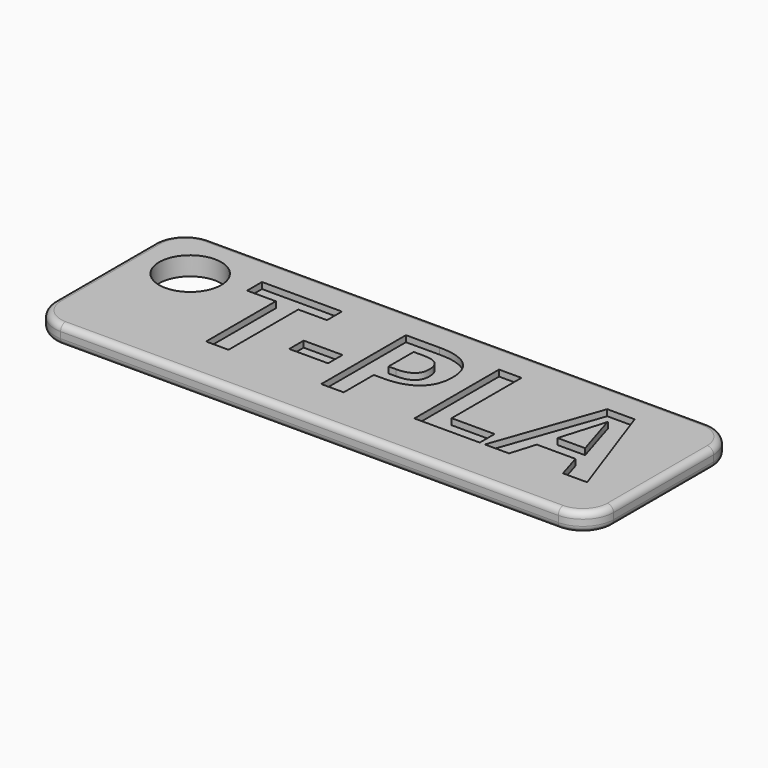
from build123d import *

# Parameters (mm, degrees)
F0_W         = 90
F0_H         = 30
F1_DEPTH     = 3
F2_R         = 1
F3_T1_DEPTH  = 3
F3_T4_ANGLE  = 90
F3_T6_ANGLE  = 90
F3_T8_ANGLE  = 90
F3_T10_ANGLE = 90
F3_T12_ANGLE = 90
F3_T14_ANGLE = 90
F3_T16_ANGLE = 90
F3_T18_ANGLE = 90
F4_R         = 5
F5_DEPTH     = 3
F6_TEXT_SIZE = 23.8714277878
F7_DEPTH     = 1


# Not quite as in the source:
# - a fillet or chamfer that OpenCascade refuses, or shapes differently, is made with other operations: its cross-section is extruded or revolved along the edge and cut away or added
# - Text() gives the source's letters only with a copy of the font that has no kerning and outlines rounded to 1/6400 em; it was checked with that copy


with BuildPart() as f1:
    # F0 (on Top) → F1 (new body)
    with BuildSketch(Plane.XY):
        Rectangle(F0_W, F0_H)
    extrude(amount=F1_DEPTH)

    # F2
    f2_edges = [f1.edges().sort_by_distance(p)[0] for p in [
        (0, 15, 3),
        (-45, 0, 3),
        (0, -15, 3),
        (45, 0, 3),
        (0, 15, 0),
        (-45, 0, 0),
        (0, -15, 0),
        (45, 0, 0),
    ]]
    fillet(f2_edges, radius=F2_R)

    # F3: fillet of radius 5 on 4 edges, made by hand

    # F3_s2 → F3_t1 (cut)
    with BuildSketch(Plane.XY):
        with BuildLine():
            ThreePointArc((45.0004, -9.9990343146), (43.5355339059, -13.5355339059), (39.9990343146, -15.0004))
            Line((39.9990343146, -15.0004), (39.9990343146, -15.5005365685))
            ThreePointArc((39.9990343146, -15.5005365685), (42.4995171573, -15.5001365685), (45, -15.5001365685))
            Line((45, -15.5001365685), (45.5001365685, -15))
            ThreePointArc((45.5001365685, -15), (45.5001365685, -12.4995171573), (45.5005365685, -9.9990343146))
            Line((45.5005365685, -9.9990343146), (45.0004, -9.9990343146))
        make_face()
        with BuildLine():
            ThreePointArc((39.9990343146, 15.0004), (43.5355339059, 13.5355339059), (45.0004, 9.9990343146))
            Line((45.0004, 9.9990343146), (45.5005365685, 9.9990343146))
            ThreePointArc((45.5005365685, 9.9990343146), (45.5001365685, 12.4995171573), (45.5001365685, 15))
            Line((45.5001365685, 15), (45, 15.5001365685))
            ThreePointArc((45, 15.5001365685), (42.4995171573, 15.5001365685), (39.9990343146, 15.5005365685))
            Line((39.9990343146, 15.5005365685), (39.9990343146, 15.0004))
        make_face()
        with BuildLine():
            ThreePointArc((-39.9990343146, 15.0004), (-43.5355339059, 13.5355339059), (-45.0004, 9.9990343146))
            Line((-45.0004, 9.9990343146), (-45.5005365685, 9.9990343146))
            ThreePointArc((-45.5005365685, 9.9990343146), (-45.5001365685, 12.4995171573), (-45.5001365685, 15))
            Line((-45.5001365685, 15), (-45, 15.5001365685))
            ThreePointArc((-45, 15.5001365685), (-42.4995171573, 15.5001365685), (-39.9990343146, 15.5005365685))
            Line((-39.9990343146, 15.5005365685), (-39.9990343146, 15.0004))
        make_face()
        with BuildLine():
            ThreePointArc((-45.0004, -9.9990343146), (-43.5355339059, -13.5355339059), (-39.9990343146, -15.0004))
            Line((-39.9990343146, -15.0004), (-39.9990343146, -15.5005365685))
            ThreePointArc((-39.9990343146, -15.5005365685), (-42.4995171573, -15.5001365685), (-45, -15.5001365685))
            Line((-45, -15.5001365685), (-45.5001365685, -15))
            ThreePointArc((-45.5001365685, -15), (-45.5001365685, -12.4995171573), (-45.5005365685, -9.9990343146))
            Line((-45.5005365685, -9.9990343146), (-45.0004, -9.9990343146))
        make_face()
    extrude(amount=F3_T1_DEPTH, mode=Mode.SUBTRACT)

    # F3_s3 → F3_t4 (revolve, cut)
    with BuildSketch(Plane.YZ.offset(-39.9990343146)):
        with BuildLine():
            ThreePointArc((-14.0004, 0), (-14.7075067812, 0.2928932188), (-15.0004, 1))
            Line((-15.0004, 1), (-15.0004, 0))
            Line((-15.0004, 0), (-14.0004, 0))
        make_face()
    revolve(axis=Axis((-39.9990343146, -9.9990343146, 0), (0, 0, -1)), revolution_arc=F3_T4_ANGLE, mode=Mode.SUBTRACT)

    # F3_s5 → F3_t6 (revolve, cut)
    with BuildSketch(Plane.XZ.offset(9.9990343146)):
        with BuildLine():
            ThreePointArc((-44.0004, 3), (-44.7075067812, 2.7071067812), (-45.0004, 2))
            Line((-45.0004, 2), (-45.0004, 3))
            Line((-45.0004, 3), (-44.0004, 3))
        make_face()
    revolve(axis=Axis((-39.9990343146, -9.9990343146, 3), (0, 0, 1)), revolution_arc=F3_T6_ANGLE, mode=Mode.SUBTRACT)

    # F3_s7 → F3_t8 (revolve, cut)
    with BuildSketch(Plane.XZ.offset(-9.9990343146)):
        with BuildLine():
            ThreePointArc((-44.0004, 0), (-44.7075067812, 0.2928932188), (-45.0004, 1))
            Line((-45.0004, 1), (-45.0004, 0))
            Line((-45.0004, 0), (-44.0004, 0))
        make_face()
    revolve(axis=Axis((-39.9990343146, 9.9990343146, 0), (0, 0, -1)), revolution_arc=F3_T8_ANGLE, mode=Mode.SUBTRACT)

    # F3_s9 → F3_t10 (revolve, cut)
    with BuildSketch(Plane.YZ.offset(-39.9990343146)):
        with BuildLine():
            ThreePointArc((14.0004, 3), (14.7075067812, 2.7071067812), (15.0004, 2))
            Line((15.0004, 2), (15.0004, 3))
            Line((15.0004, 3), (14.0004, 3))
        make_face()
    revolve(axis=Axis((-39.9990343146, 9.9990343146, 3), (0, 0, 1)), revolution_arc=F3_T10_ANGLE, mode=Mode.SUBTRACT)

    # F3_s11 → F3_t12 (revolve, cut)
    with BuildSketch(Plane.YZ.offset(39.9990343146)):
        with BuildLine():
            ThreePointArc((14.0004, 0), (14.7075067812, 0.2928932188), (15.0004, 1))
            Line((15.0004, 1), (15.0004, 0))
            Line((15.0004, 0), (14.0004, 0))
        make_face()
    revolve(axis=Axis((39.9990343146, 9.9990343146, 0), (0, 0, -1)), revolution_arc=F3_T12_ANGLE, mode=Mode.SUBTRACT)

    # F3_s13 → F3_t14 (revolve, cut)
    with BuildSketch(Plane.XZ.offset(-9.9990343146)):
        with BuildLine():
            ThreePointArc((44.0004, 3), (44.7075067812, 2.7071067812), (45.0004, 2))
            Line((45.0004, 2), (45.0004, 3))
            Line((45.0004, 3), (44.0004, 3))
        make_face()
    revolve(axis=Axis((39.9990343146, 9.9990343146, 3), (0, 0, 1)), revolution_arc=F3_T14_ANGLE, mode=Mode.SUBTRACT)

    # F3_s15 → F3_t16 (revolve, cut)
    with BuildSketch(Plane.XZ.offset(9.9990343146)):
        with BuildLine():
            ThreePointArc((44.0004, 0), (44.7075067812, 0.2928932188), (45.0004, 1))
            Line((45.0004, 1), (45.0004, 0))
            Line((45.0004, 0), (44.0004, 0))
        make_face()
    revolve(axis=Axis((39.9990343146, -9.9990343146, 0), (0, 0, -1)), revolution_arc=F3_T16_ANGLE, mode=Mode.SUBTRACT)

    # F3_s17 → F3_t18 (revolve, cut)
    with BuildSketch(Plane.YZ.offset(39.9990343146)):
        with BuildLine():
            ThreePointArc((-14.0004, 3), (-14.7075067812, 2.7071067812), (-15.0004, 2))
            Line((-15.0004, 2), (-15.0004, 3))
            Line((-15.0004, 3), (-14.0004, 3))
        make_face()
    revolve(axis=Axis((39.9990343146, -9.9990343146, 3), (0, 0, 1)), revolution_arc=F3_T18_ANGLE, mode=Mode.SUBTRACT)

    # F4 (on face) → F5 (cut)
    with BuildSketch(Plane.XY.offset(3)):
        with Locations((-36, 6)):
            Circle(F4_R)
    extrude(amount=-F5_DEPTH, mode=Mode.SUBTRACT)

    # F6 (on face) → F7 (cut)
    with BuildSketch(Plane.XY.offset(3)):
        with Locations((-28, -7.1874280072)):
            Text('T-PLA', F6_TEXT_SIZE, font='Open Sans', font_style=FontStyle.BOLD, text_align=(TextAlign.LEFT, TextAlign.BOTTOM))
    extrude(amount=-F7_DEPTH, mode=Mode.SUBTRACT)


solid = f1.part
